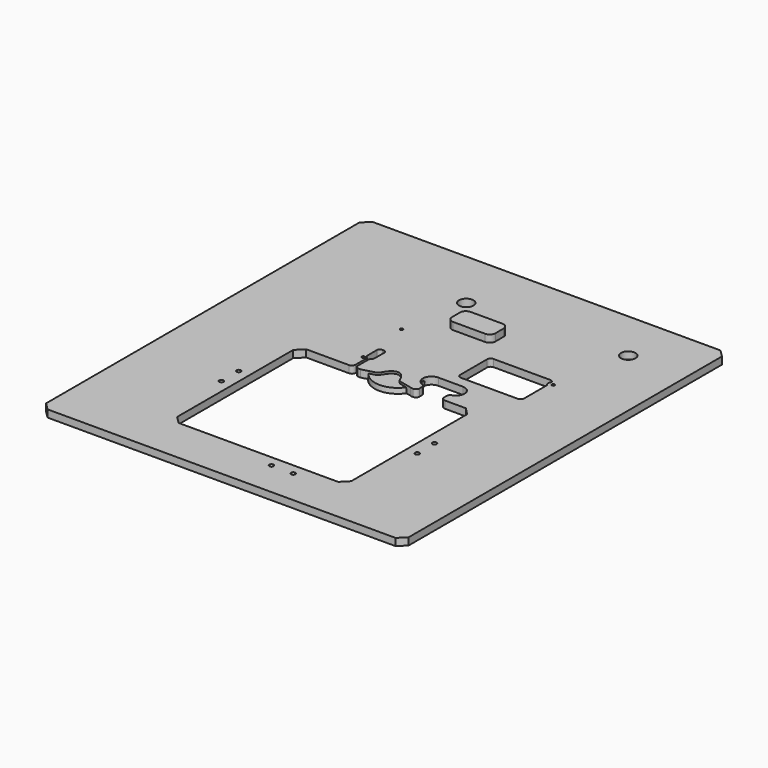
from build123d import *

# Parameters (mm, degrees)
F1_W     = 500
F1_H     = 560
F1_R     = 3
F1_R_2   = 2
F1_R_3   = 10
F2_DEPTH = 10
F4_DEPTH = 10
F5_SIZE  = 10


with BuildPart() as f2:
    # F1 (on Top) → F2 (new body)
    with BuildSketch(Plane.XY):
        with Locations((0, -23.7707149982)):
            Rectangle(F1_W, F1_H)
        with Locations((30.0772486633, -255.3247647732)):
            Circle(F1_R, mode=Mode.SUBTRACT)
        with Locations((60.0772486633, -255.3247647732)):
            Circle(F1_R, mode=Mode.SUBTRACT)
        with Locations((-135, -135.3247647732)):
            Circle(F1_R, mode=Mode.SUBTRACT)
        with Locations((-135, -105.3247647732)):
            Circle(F1_R, mode=Mode.SUBTRACT)
        with Locations((-50.876, 3.837)):
            Circle(F1_R_2, mode=Mode.SUBTRACT)
        with Locations((-58.876, 80.337)):
            Circle(F1_R_2, mode=Mode.SUBTRACT)
        with Locations((-43.0248305202, 171.7090308666)):
            Circle(F1_R_3, mode=Mode.SUBTRACT)
        with BuildLine():
            Line((-120, -240.3247647732), (-120, -20.3247647732))
            Line((-120, -20.3247647732), (-51.0308213367, -20.3247647732))
            ThreePointArc((-51.0308213367, -20.3247647732), (-47.4952874307, -18.8602986792), (-46.0308213367, -15.3247647732))
            Line((-46.0308213367, -15.3247647732), (-46.0308213367, 2.308832501))
            ThreePointArc((-46.0308213367, 2.308832501), (-46.5016989751, 4.4270984509), (-47.8256415904, 6.1463867735))
            ThreePointArc((-47.8256415904, 6.1463867735), (-48.9637284761, 7.5993782677), (-49.4086683367, 9.3905942128))
            Line((-49.4086683367, 9.3905942128), (-49.4086683367, 25.6183712128))
            ThreePointArc((-49.4086683367, 25.6183712128), (-48.0654966834, 28.6648038331), (-44.9548493367, 29.8517052128))
            Line((-44.9548493367, 29.8517052128), (-43.7678212187, 29.8517052128))
            ThreePointArc((-43.7678212187, 29.8517052128), (-40.637428861, 28.6788851912), (-39.2927663367, 25.6183712128))
            Line((-39.2927663367, 25.6183712128), (-39.2927663367, 9.3905942128))
            ThreePointArc((-39.2927663367, 9.3905942128), (-39.7377071117, 7.5993718655), (-40.8757968434, 6.1463744279))
            ThreePointArc((-40.8757968434, 6.1463744279), (-42.1997367361, 4.4270870271), (-42.6706133367, 2.3088232963))
            Line((-42.6706133367, 2.3088232963), (-42.6706133367, -15.3247647732))
            ThreePointArc((-42.6706133367, -15.3247647732), (-41.2061472426, -18.8602986792), (-37.6706133367, -20.3247647732))
            Line((-37.6706133367, -20.3247647732), (-35.1419784129, -20.3247647732))
            add(Edge.make_bspline(
                [(-35.1419784129, -20.3247647732), (-34.1598968907, -19.9685891101), (-31.3607001601, -19.6192307571), (-29.8467303867, -18.8231529819), (-27.7683977823, -18.3917721381), (-26.3336397017, -18.0135299785), (-22.5796525571, -17.0853870147), (-18.9456036242, -16.0671039066), (-16.7320655768, -15.5646387194), (-14.8111856629, -14.16932632), (-13.3695590782, -12.1752079912), (-12.2022525833, -9.7286932544), (-11.491348561, -8.7693558731), (-10.3865304992, -6.8674624113), (-6.8191670577, -2.3486430291), (-3.6730417858, -1.0682009745), (-0.0323925139, 0.4933333957), (3.8484487001, -0.8160184171), (6.2819386152, -2.3766355402), (8.2280909316, -4.3878710315), (10.3123406285, -7.0470809276), (11.2202460098, -8.8079307876), (12.3250038703, -10.7817132124), (13.3005723278, -12.9605031724), (14.3129998399, -15.4180110053), (19.9388190144, -16.5153375349), (24.2851598431, -17.7430543029), (28.8066153808, -18.5117694503), (33.3233263839, -19.6542728052), (34.1151070689, -20.1492249102), (34.3248918653, -20.3247647732)],
                knots=[0, 0, 0, 0, 0.0406361494, 0.0690843533, 0.0982832849, 0.1240792745, 0.1650586975, 0.2064474949, 0.237602636, 0.2688839918, 0.3023509551, 0.3363941823, 0.3586454287, 0.3892430987, 0.4390503332, 0.478234315, 0.5186842811, 0.5600640859, 0.5954673894, 0.6306059239, 0.6688365072, 0.6984296576, 0.7295419634, 0.7618620205, 0.7940667479, 0.8425634492, 0.8880772951, 0.9338149024, 0.9784648643, 1, 1, 1, 1], degree=3))
            Line((34.3248918653, -20.3247647732), (37.3092798889, -20.3247647732))
            ThreePointArc((37.3092798889, -20.3247647732), (40.8448137948, -18.8602986792), (42.3092798889, -15.3247647732))
            Line((42.3092798889, -15.3247647732), (42.3092798889, -10.7997291517))
            ThreePointArc((42.3092798889, -10.7997291517), (41.3371476596, -7.8372502536), (38.7987674003, -6.0267398417))
            ThreePointArc((38.7987674003, -6.0267398417), (30.6595093232, 6.9980494805), (42.3092798889, 17.0068208687))
            Line((42.3092798889, 17.0068208687), (76.0486274958, 17.0068208687))
            ThreePointArc((76.0486274958, 17.0068208687), (87.6983980614, 6.9980494805), (79.5591399843, -6.0267398417))
            ThreePointArc((79.5591399843, -6.0267398417), (77.020759725, -7.8372502536), (76.0486274958, -10.7997291517))
            Line((76.0486274958, -10.7997291517), (76.0486274958, -15.3247647732))
            ThreePointArc((76.0486274958, -15.3247647732), (77.5130935898, -18.8602986792), (81.0486274958, -20.3247647732))
            Line((81.0486274958, -20.3247647732), (120, -20.3247647732))
            Line((120, -20.3247647732), (120, -240.3247647732))
            Line((120, -240.3247647732), (-120, -240.3247647732))
        make_face(mode=Mode.SUBTRACT)
        with Locations((135, -135.3247647732)):
            Circle(F1_R, mode=Mode.SUBTRACT)
        with Locations((135, -105.3247647732)):
            Circle(F1_R, mode=Mode.SUBTRACT)
        with BuildLine():
            ThreePointArc((56.6810779274, 83.0211144686), (58.1455440214, 86.5566483745), (61.6810779274, 88.0211144686))
            Line((61.6810779274, 88.0211144686), (139.8661386967, 88.0211144686))
            ThreePointArc((139.8661386967, 88.0211144686), (142.5837054983, 87.2181170512), (144.4283926506, 85.0670467401))
            ThreePointArc((144.4283926506, 85.0670467401), (142.9093529183, 80.513034466), (144.8661386967, 76.129257679))
            Line((144.8661386967, 76.129257679), (144.8661386967, 36.8050682545))
            ThreePointArc((144.8661386967, 36.8050682545), (143.4016726026, 33.2695343485), (139.8661386967, 31.8050682545))
            Line((139.8661386967, 31.8050682545), (61.6810779274, 31.8050682545))
            ThreePointArc((61.6810779274, 31.8050682545), (58.1455440214, 33.2695343485), (56.6810779274, 36.8050682545))
            Line((56.6810779274, 36.8050682545), (56.6810779274, 83.0211144686))
        make_face(mode=Mode.SUBTRACT)
        with Locations((149.524, 80.837)):
            Circle(F1_R_2, mode=Mode.SUBTRACT)
        with Locations((169.9751694798, 184.7090308666)):
            Circle(F1_R_3, mode=Mode.SUBTRACT)
    extrude(amount=F2_DEPTH)

    # F5
    f5_edges = [f2.edges().sort_by_distance(p)[0] for p in [
        (-120, -20.324765, 5),
        (120, -20.324765, 5),
        (120, -240.324765, 5),
        (-120, -240.324765, 5),
        (250, -303.770715, 5),
        (250, 256.229285, 5),
        (-250, 256.229285, 5),
        (-250, -303.770715, 5),
    ]]
    chamfer(f5_edges, length=F5_SIZE)


with BuildPart() as f4:
    # F3 (on face) → F4 (new body)
    with BuildSketch(Plane.XY.offset(10)):
        with BuildLine():
            ThreePointArc((37.7411322854, 135.2619925924), (35.3979865349, 140.9188468419), (29.7411322854, 143.2619925924))
            Line((29.7411322854, 143.2619925924), (-14.2588677146, 143.2619925924))
            ThreePointArc((-14.2588677146, 143.2619925924), (-19.915721964, 140.9188468419), (-22.2588677146, 135.2619925924))
            Line((-22.2588677146, 135.2619925924), (-22.2588677146, 121.2619925924))
            ThreePointArc((-22.2588677146, 121.2619925924), (-19.915721964, 115.6051383429), (-14.2588677146, 113.2619925924))
            Line((-14.2588677146, 113.2619925924), (29.7411322854, 113.2619925924))
            ThreePointArc((29.7411322854, 113.2619925924), (35.3979865349, 115.6051383429), (37.7411322854, 121.2619925924))
            Line((37.7411322854, 121.2619925924), (37.7411322854, 135.2619925924))
        make_face()
    extrude(amount=F4_DEPTH)


with BuildPart() as f7:
    # F6 (on Right) → F7 (revolve)
    with BuildSketch(Plane.YZ):
        Polygon((0, 7), (0, 0), (32, 0), (31.5, 7), align=None)
    revolve(axis=Axis((0, 0, 3.5), (0, 0, -1)))


solid = Compound([f2.part, f4.part, f7.part])
